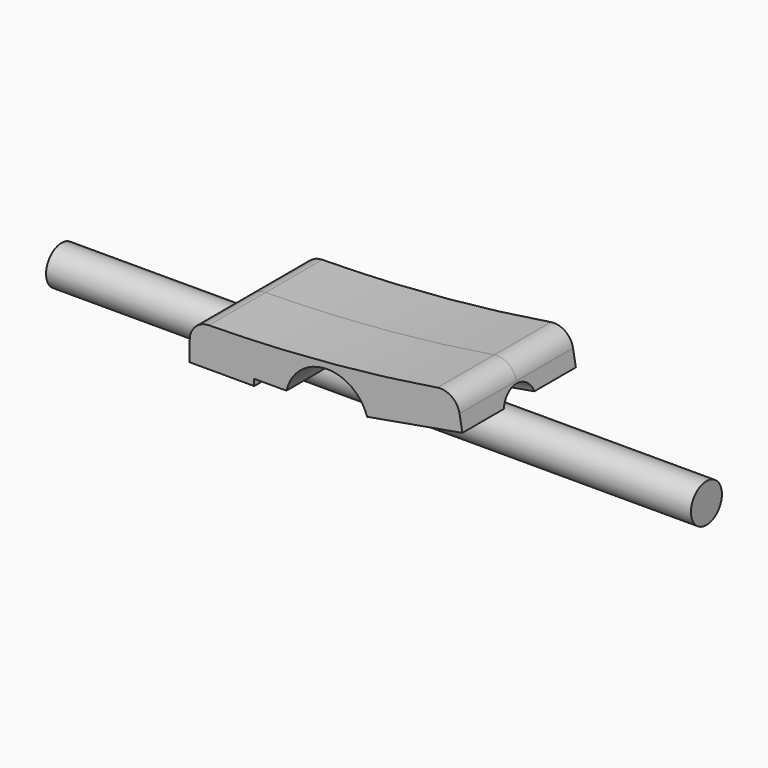
from build123d import *

# Parameters (mm, degrees)
F1_DEPTH = 11
F2_R     = 3.1
F3_DEPTH = 30
F5_DEPTH = 60
F6_R     = 3
F7_DEPTH = 50
F8_R     = 3.55
F8_R_2   = 2.25
F9_DEPTH = 2
F11_R    = 3


# Not quite as in the source:
# - a fillet or chamfer that OpenCascade refuses, or shapes differently, is made with other operations: its cross-section is extruded or revolved along the edge and cut away or added


with BuildPart() as f1:
    # F0 (on Front) → F1 (new body, symmetric)
    with BuildSketch(Plane.XZ):
        with BuildLine():
            Line((-11.3245553203, 1.5), (-6.3245553203, 1.5))
            ThreePointArc((-6.3245553203, 1.5), (-4.0311288741, 5.0990195136), (0, 6.5))
            Line((0, 6.5), (-21.3245553203, 6.5))
            Line((-21.3245553203, 6.5), (-21.3245553203, 0.5))
            Line((-21.3245553203, 0.5), (-11.3245553203, 0.5))
            Line((-11.3245553203, 0.5), (-11.3245553203, 1.5))
        make_face()
        with BuildLine():
            ThreePointArc((0, 6.5), (3.8219824935, 5.2576087549), (6.182919575, 2.0053691753))
            Line((6.182919575, 2.0053691753), (20.9550358702, 4.6100918403))
            Line((20.9550358702, 4.6100918403), (19.999970893, 10.0265344818))
            Line((19.999970893, 10.0265344818), (0, 6.5))
        make_face()
        with BuildLine():
            Line((-21.3245553203, 6.5), (0, 6.5))
            Line((0, 6.5), (19.999970893, 10.0265344818))
            add(Edge.make_bspline(
                [(19.999970893, 10.0265344818), (6.3930427733, 7.6272659298), (-7.5069618116, 6.5), (-21.3245553203, 6.5)],
                knots=[0, 0, 0, 0, 41.4747261861, 41.4747261861, 41.4747261861, 41.4747261861], degree=3))
        make_face()
    extrude(amount=F1_DEPTH, both=True)

    # F2 (on Right) → F3 (cut, symmetric)
    with BuildSketch(Plane.YZ):
        Circle(F2_R)
    extrude(amount=F3_DEPTH, both=True, mode=Mode.SUBTRACT)

    # F4 (on face) → F5 (cut)
    with BuildSketch(Plane(origin=(21.1115363588, 0, 3.7225334643), x_dir=(0, 1, 0), z_dir=(0.984807753, 0, 0.1736481777))):
        with BuildLine():
            Line((-2.9660997499, 0.9012503946), (2.9660997499, 0.9012503946))
            ThreePointArc((2.9660997499, 0.9012503946), (0, 3.1), (-2.9660997499, 0.9012503946))
        make_face()
        with BuildLine():
            ThreePointArc((-2.9660997499, 0.9012503946), (-0.4555714957, -3.0663422204), (3.1, 0))
            ThreePointArc((3.1, 0), (3.0663422204, 0.4555714957), (2.9660997499, 0.9012503946))
            Line((2.9660997499, 0.9012503946), (-2.9660997499, 0.9012503946))
        make_face()
    extrude(amount=-F5_DEPTH, mode=Mode.SUBTRACT)

    # F8 (on face) → F9 (cut)
    with BuildSketch(Plane(origin=(-0.1565004886, 0, 0.887558376), x_dir=(0.984807753, 0, 0.1736481777), z_dir=(0.1736481777, 0, -0.984807753))):
        with Locations((16.4372158365, 6.9830498749)):
            Circle(F8_R)
        with Locations((16.4372158365, 6.9830498749)):
            Circle(F8_R_2, mode=Mode.SUBTRACT)
        with Locations((16.4372158365, -6.9830498749)):
            Circle(F8_R)
        with Locations((16.4372158365, -6.9830498749)):
            Circle(F8_R_2, mode=Mode.SUBTRACT)
    extrude(amount=-F9_DEPTH, mode=Mode.SUBTRACT)

    # F10: chamfer of 2 on 2 edges, made by hand


with BuildPart() as f7:
    # F6 (on Right) → F7 (new body, symmetric)
    with BuildSketch(Plane.YZ):
        Circle(F6_R)
    extrude(amount=F7_DEPTH, both=True)


with BuildPart() as f10_tool2:
    # F10_s3 → F10_t4 (revolve)
    with BuildSketch(Plane.XZ.offset(6.9830498749)):
        Polygon((17.8995181941, 6.1021748577), (16.2771990434, 3.7852629963), (18.2468145494, 4.1325593517), align=None)
    revolve(axis=Axis((16.0309971051, -6.9830498749, 3.7418509519), (0.1736481777, 0, -0.984807753)))

    split(bisect_by=Plane(origin=(-0.503796844, 0, 2.857173882), x_dir=(0, 1, 0), z_dir=(0.1736481777, 0, -0.984807753)), keep=Keep.TOP)


with BuildPart() as f1_1:
    add(f1.part)

    # F10_t1: cut F10_tool2
    add(f10_tool2.part, mode=Mode.SUBTRACT)


with BuildPart() as f10_tool7:
    # F10_s8 → F10_t9 (revolve)
    with BuildSketch(Plane.XZ.offset(-6.9830498749)):
        Polygon((17.8995181941, 6.1021748577), (16.2771990434, 3.7852629963), (18.2468145494, 4.1325593517), align=None)
    revolve(axis=Axis((16.0309971051, 6.9830498749, 3.7418509519), (0.1736481777, 0, -0.984807753)))

    split(bisect_by=Plane(origin=(-0.503796844, 0, 2.857173882), x_dir=(0, 1, 0), z_dir=(0.1736481777, 0, -0.984807753)), keep=Keep.TOP)


with BuildPart() as f1_2:
    add(f1_1.part)

    # F10_t6: cut F10_tool7
    add(f10_tool7.part, mode=Mode.SUBTRACT)

    # F11
    f11_edges = [f1_2.edges().sort_by_distance(p)[0] for p in [
        (19.999971, -5.5, 10.026534),
        (19.999971, 5.5, 10.026534),
        (-21.324555, -5.5, 6.5),
        (-21.324555, 5.5, 6.5),
    ]]
    fillet(f11_edges, radius=F11_R)


solid = Compound([f7.part, f1_2.part])
